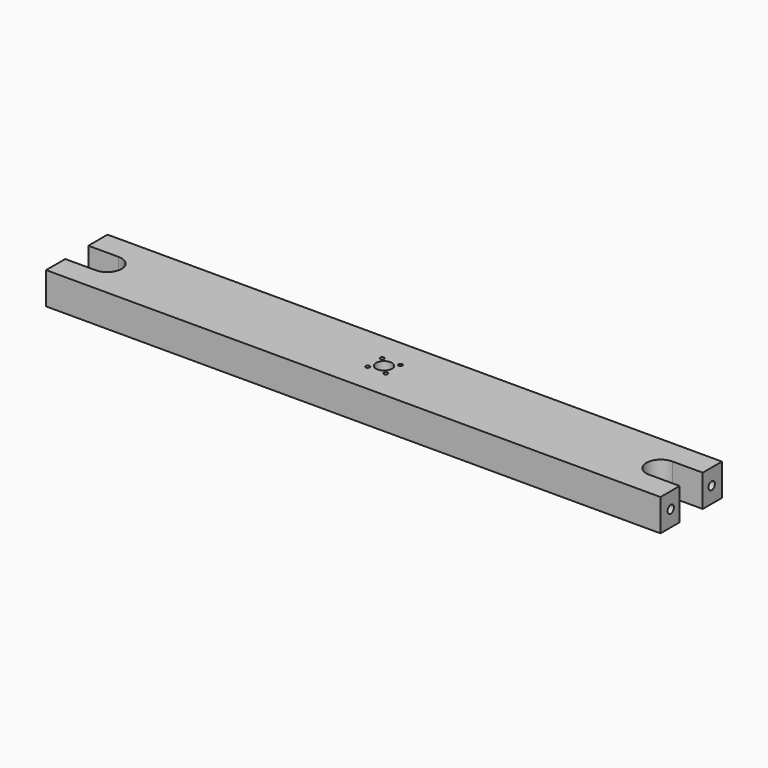
from build123d import *

# Parameters (mm, degrees)
F1_DEPTH = 20
F2_R     = 2.5
F3_DEPTH = 25
F4_R     = 5
F4_R_2   = 1.25
F5_DEPTH = 25


# Not quite as in the source:
# - a pattern or mirror of a feature is missing from the dataset's text; its kind, count and spacing are read off the source's solid


with BuildPart() as f1:
    # F0 (on Top) → F1 (new body)
    with BuildSketch(Plane.XY):
        with BuildLine():
            Line((-192, -24), (192, -24))
            Line((192, -24), (192, -9))
            Line((192, -9), (173, -9))
            ThreePointArc((173, -9), (164, 0), (173, 9))
            Line((173, 9), (192, 9))
            Line((192, 9), (192, 24))
            Line((192, 24), (-192, 24))
            Line((-192, 24), (-192, 9))
            Line((-192, 9), (-173, 9))
            ThreePointArc((-173, 9), (-164, 0), (-173, -9))
            Line((-173, -9), (-192, -9))
            Line((-192, -9), (-192, -24))
        make_face()
    extrude(amount=F1_DEPTH)

    # F2 (on face) → F3 (cut)
    with BuildSketch(Plane(origin=(-192, 0, 0), x_dir=(0, -1, 0), z_dir=(-1, 0, 0))):
        with Locations((-16, 10)):
            Circle(F2_R)
        with Locations((16, 10)):
            Circle(F2_R)
    f3 = extrude(amount=-F3_DEPTH, mode=Mode.SUBTRACT)

    # F3_copies: F3 across plane
    add(f3.mirror(Plane(origin=(0, 0, 0), x_dir=(0, 0, 1), z_dir=(1, 0, 0))), mode=Mode.SUBTRACT)

    # F4 (on face) → F5 (cut)
    with BuildSketch(Plane(origin=(0, 0, 0), x_dir=(1, 0, 0), z_dir=(0, 0, -1))):
        Circle(F4_R)
        with Locations((-5.6568542495, 5.6568542495)):
            Circle(F4_R_2)
        with Locations((-5.6568542495, -5.6568542495)):
            Circle(F4_R_2)
        with Locations((5.6568542495, -5.6568542495)):
            Circle(F4_R_2)
        with Locations((5.6568542495, 5.6568542495)):
            Circle(F4_R_2)
    extrude(amount=-F5_DEPTH, mode=Mode.SUBTRACT)


solid = f1.part
